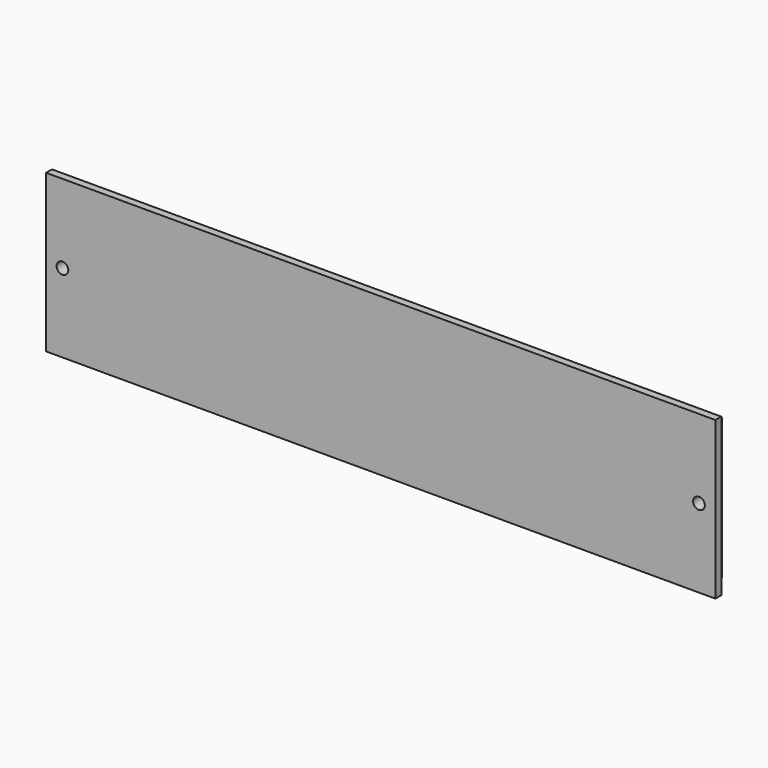
from build123d import *

# Parameters (mm, degrees)
F0_W     = 159.4
F0_H     = 34.4
F0_R     = 1.425
F1_DEPTH = 4.5
F0_W_2   = 163.4
F0_H_2   = 38.4
F2_DEPTH = 1.8


with BuildPart() as f1:
    # F0 (on Front) → F1 (new body)
    with BuildSketch(Plane.XZ):
        Rectangle(F0_W, F0_H)
        with Locations((-77.7, 0)):
            Circle(F0_R, mode=Mode.SUBTRACT)
        with Locations((77.7, 0)):
            Circle(F0_R, mode=Mode.SUBTRACT)
    extrude(amount=-F1_DEPTH)

    # F0 (on Front) → F2 (join)
    with BuildSketch(Plane.XZ):
        Rectangle(F0_W_2, F0_H_2)
        Rectangle(F0_W, F0_H, mode=Mode.SUBTRACT)
    extrude(amount=-F2_DEPTH)


solid = f1.part
